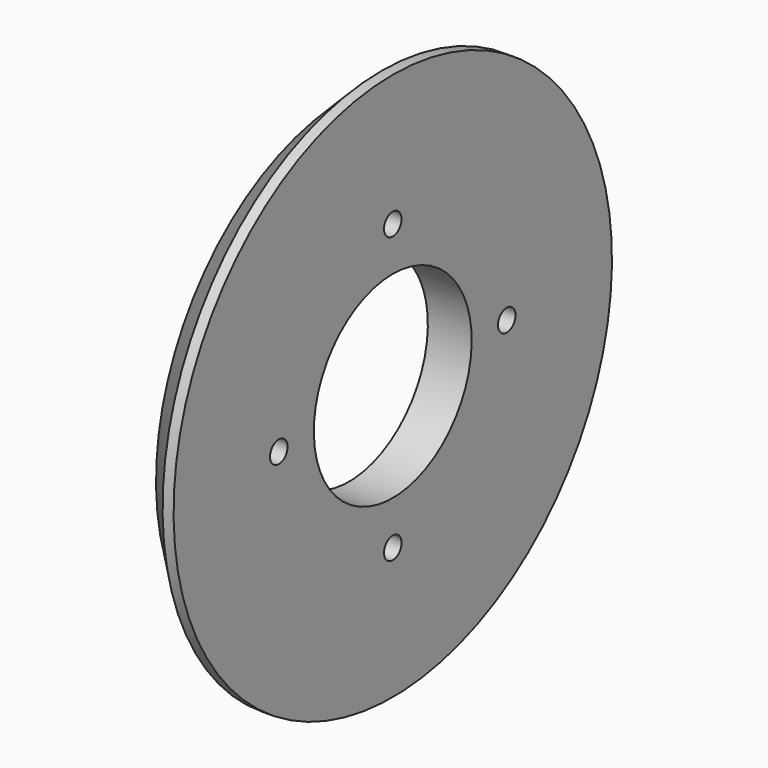
from build123d import *

# Parameters (mm, degrees)
F3_D            = 2
F3_DEPTH        = 4
F3_CBORE_D      = 4.4
F3_CBORE_DEPTH  = 2
F3_TIP          = 0.600860619
F3_COPIES_COUNT = 4


# Not quite as in the source:
# - a pattern or mirror of a feature is missing from the dataset's text; its kind, count and spacing are read off the source's solid


with BuildPart() as f1:
    # F0 (on Front) → F1 (revolve)
    with BuildSketch(Plane.XZ):
        Polygon((-4, 9), (0, 9), (0, 25), (-1, 25), (-4, 22), align=None)
    revolve(axis=Axis((-2, 0, 0), (1, 0, 0)))

    # F3
    with Locations(Plane(origin=(-4, 0, 0), x_dir=(0, -1, 0), z_dir=(-1, 0, 0))):
        with Locations((0, 13)):
            f3 = CounterBoreHole(F3_D / 2, F3_CBORE_D / 2, F3_CBORE_DEPTH, depth=F3_DEPTH)
            with Locations((0, 0, -(F3_DEPTH + F3_TIP / 2))):  # 118° drill point
                Cone(0, F3_D / 2, F3_TIP, mode=Mode.SUBTRACT)

    # F3_copies: F3 ×4 about axis
    f3_copies_axis = Axis((0, 0, 0), (1, 0, 0))
    for i in range(1, F3_COPIES_COUNT):
        add(f3.rotate(f3_copies_axis, i * 360 / F3_COPIES_COUNT), mode=Mode.SUBTRACT)


solid = f1.part
